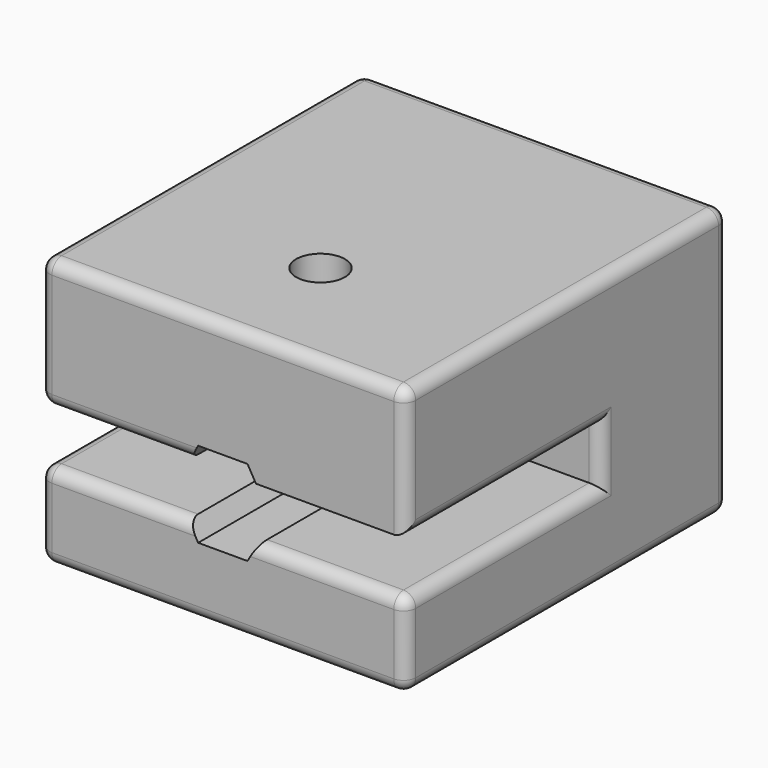
from build123d import *

# Parameters (mm, degrees)
F0_W          = 30
F0_H          = 33
F1_DEPTH      = 22
F2_W          = 20
F2_H          = 4.4
F3_DEPTH      = 30.001
F4_R          = 2
F5_DEPTH      = 5
F5_DEPTH_BACK = 20.001
F6_DEPTH      = 13.001
F7_R          = 2
F8_DEPTH      = 10.601
F9_DEPTH      = 3.5
F10_R         = 1


with BuildPart() as f1:
    # F0 (on Top) → F1 (new body)
    with BuildSketch(Plane.XY):
        Rectangle(F0_W, F0_H)
    extrude(amount=F1_DEPTH)

    # F2 (on face) → F3 (cut, through all)
    with BuildSketch(Plane.YZ.offset(15)):
        with Locations((-6.5, 9.2)):
            Rectangle(F2_W, F2_H)
    extrude(amount=-F3_DEPTH, mode=Mode.SUBTRACT)

    # F4 (on face) → F5 (cut, two sides)
    with BuildSketch(Plane.XZ.offset(-3.5)) as f5_sk:
        Polygon((-2.7135462652, 11.4), (2.7135462652, 11.4), (2.0207259422, 12.6), (-2.0207259422, 12.6), align=None)
        Polygon((-2.829016319, 7), (2.829016319, 7), (4.0414518843, 9.1), (2.7135462652, 11.4), (-2.7135462652, 11.4), (-4.0414518843, 9.1), align=None)
        with Locations((0, 9.1)):
            Circle(F4_R, mode=Mode.SUBTRACT)
        Polygon((-2.0207259422, 5.6), (2.0207259422, 5.6), (2.829016319, 7), (-2.829016319, 7), align=None)
    extrude(amount=-F5_DEPTH, mode=Mode.SUBTRACT)
    extrude(f5_sk.sketch, amount=F5_DEPTH_BACK, mode=Mode.SUBTRACT)

    # F6 (cut, through all): a face of the model
    f6_faces = [f1.faces().sort_by_distance(p)[0] for p in [
        (0, 3.5, 9.1),
    ]]
    extrude(f6_faces, amount=-F6_DEPTH, mode=Mode.SUBTRACT)

    # F7 (on face) → F8 (cut, through all)
    with BuildSketch(Plane(origin=(0, 0, 11.4), x_dir=(1, 0, 0), z_dir=(0, 0, -1))):
        with Locations((0, 6.5)):
            Circle(F7_R)
    extrude(amount=-F8_DEPTH, mode=Mode.SUBTRACT)

    # F7 (on face) → F9 (cut)
    with BuildSketch(Plane(origin=(0, 0, 11.4), x_dir=(1, 0, 0), z_dir=(0, 0, -1))):
        Polygon((-4.0414518843, 6.5), (-2.7135462652, 4.2), (-2.7135462652, 8.8), align=None)
        Polygon((-2.7135462652, 8.8), (-2.7135462652, 4.2), (-2.0207259422, 3), (2.0207259422, 3), (2.7135462652, 4.2), (2.7135462652, 8.8), (2.0207259422, 10), (-2.0207259422, 10), align=None)
        with Locations((0, 6.5)):
            Circle(F7_R, mode=Mode.SUBTRACT)
        Polygon((2.7135462652, 8.8), (2.7135462652, 4.2), (4.0414518843, 6.5), align=None)
    extrude(amount=-F9_DEPTH, mode=Mode.SUBTRACT)

    # F10
    f10_edges = [f1.edges().sort_by_distance(p)[0] for p in [
        (0, 16.5, 0),
        (15, 16.5, 11),
        (0, 16.5, 22),
        (-15, 16.5, 11),
        (-15, 0, 0),
        (0, -16.5, 0),
        (15, 0, 0),
        (-15, 0, 22),
        (0, -16.5, 22),
        (15, 0, 22),
        (-15, -16.5, 3.5),
        (-15, -16.5, 16.7),
        (15, -16.5, 3.5),
        (15, -16.5, 16.7),
        (15, -6.5, 11.4),
        (15, -6.5, 7),
        (8.914508, -16.5, 7),
        (-8.914508, -16.5, 7),
        (-8.856773, -16.5, 11.4),
        (-15, 3.5, 9.2),
        (-15, -6.5, 7),
        (-15, -6.5, 11.4),
        (15, 3.5, 9.2),
    ]]
    fillet(f10_edges, radius=F10_R)


solid = f1.part
